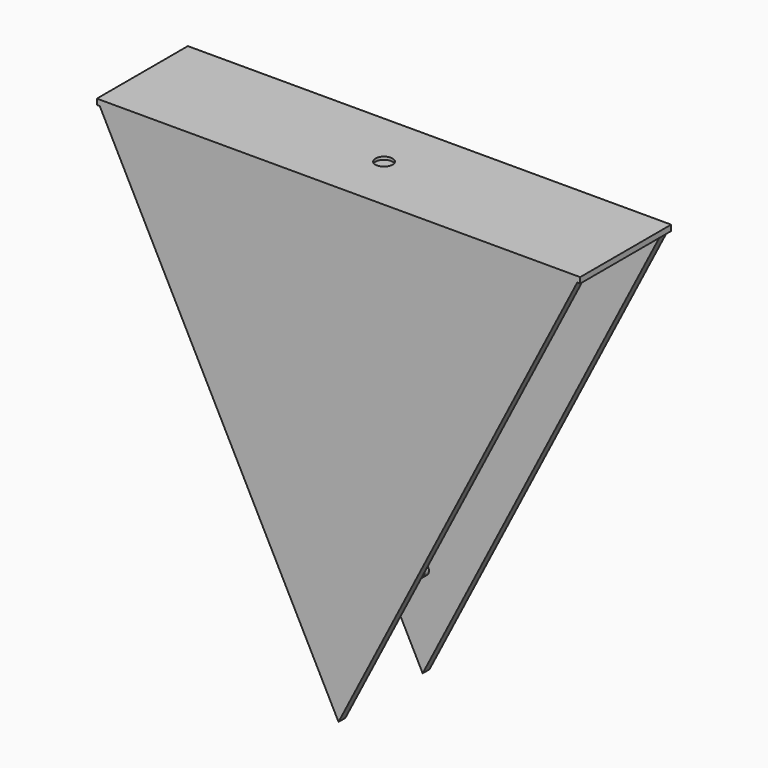
from build123d import *

# Parameters (mm, degrees)
F0_W      = 170
F0_H      = 34
F1_DEPTH  = 2
F2_W      = 170
F2_H      = 2
F4_DEPTH  = 3
F5_W      = 170
F5_H      = 2
F7_DEPTH  = 3
F8_R      = 2
F9_DEPTH  = 2
F10_R     = 1
F11_DEPTH = 1
F12_R     = 3
F13_DEPTH = 1


with BuildPart() as f1:
    # F0 (on Top) → F1 (new body)
    with BuildSketch(Plane.XY):
        with Locations((-8.2408198714, -30.0435358584)):
            Rectangle(F0_W, F0_H)
    extrude(amount=F1_DEPTH)

    # F2 (on face) + F3 (on face) → F4 (join)
    with BuildSketch(Plane.XZ.offset(47.0435358584)):
        with Locations((-8.2408198714, 1)):
            Rectangle(F2_W, F2_H)
    with BuildSketch(Plane.XZ.offset(47.0435358584)):
        Polygon((75.7311444739, 0), (-92.2127468976, 0), (-8.2416068763, -163.3778810501), align=None)
    extrude(amount=F4_DEPTH)

    # F6 (on face) + F5 (on face) → F7 (join)
    with BuildSketch(Plane(origin=(0, -13.0435358584, 0), x_dir=(-1, 0, 0), z_dir=(0, 1, 0))):
        Polygon((92.2128885412, 0), (-75.7311794344, 0), (8.2415537909, -163.3778512478), align=None)
    with BuildSketch(Plane(origin=(0, -13.0435358584, 0), x_dir=(-1, 0, 0), z_dir=(0, 1, 0))):
        with Locations((8.2408198714, 1)):
            Rectangle(F5_W, F5_H)
    extrude(amount=F7_DEPTH)

    # F8 (on face) → F9 (join)
    with BuildSketch(Plane.XZ.offset(13.0435358584)):
        with Locations((-8.0062086027, -130.911280853)):
            Circle(F8_R)
    extrude(amount=F9_DEPTH)

    # F10 (on face) → F11 (cut)
    with BuildSketch(Plane.XZ.offset(15.0435358584)):
        with Locations((-8.0062086027, -130.911280853)):
            Circle(F10_R)
    extrude(amount=-F11_DEPTH, mode=Mode.SUBTRACT)

    # F12 (on face) → F13 (cut)
    with BuildSketch(Plane.XY.offset(2)):
        with Locations((-8.2408198714, -30.0435358584)):
            Circle(F12_R)
    extrude(amount=-F13_DEPTH, mode=Mode.SUBTRACT)


solid = f1.part
